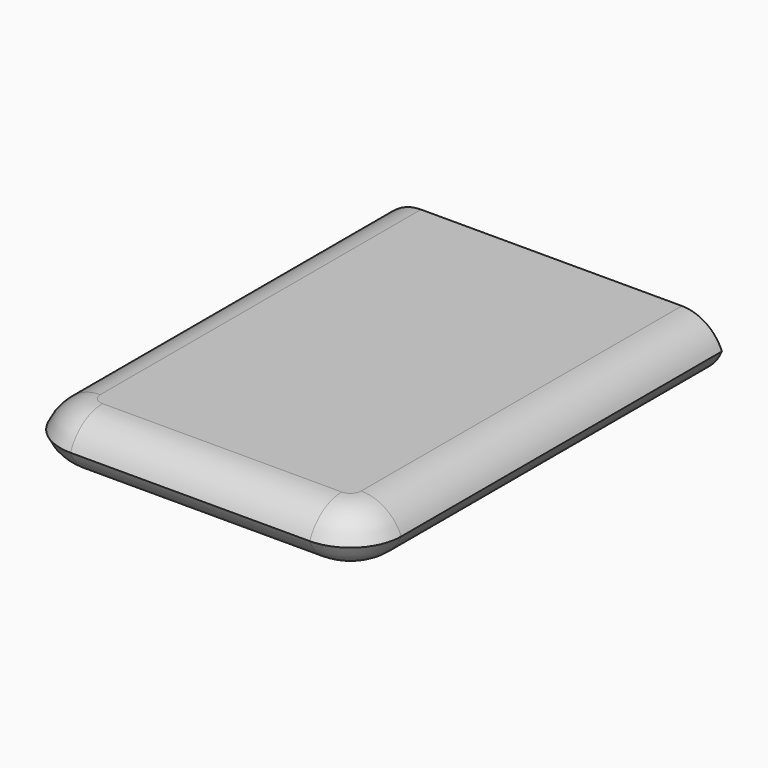
from build123d import *

# Parameters (mm, degrees)
F1_DEPTH     = 6.35
F2_T1_DEPTH  = 59.8574546933
F2_T3_DEPTH  = 28.1503971994
F2_T6_ANGLE  = 90
F2_T8_ANGLE  = 90
F2_T10_ANGLE = 90
F2_T12_ANGLE = 90


# Not quite as in the source:
# - a fillet or chamfer that OpenCascade refuses, or shapes differently, is made with other operations: its cross-section is extruded or revolved along the edge and cut away or added


with BuildPart() as f1:
    # F0 (on Top) → F1 (new body)
    with BuildSketch(Plane.XY):
        with BuildLine():
            Line((20.4174276441, 0), (-20.4329695553, 0))
            Line((-20.4329695553, 0), (-20.4329695553, -47.1574546933))
            ThreePointArc((-20.4329695553, -47.1574546933), (-18.5730976158, -51.6475827539), (-14.0829695553, -53.5074546933))
            Line((-14.0829695553, -53.5074546933), (14.0674276441, -53.5074546933))
            ThreePointArc((14.0674276441, -53.5074546933), (18.5575557047, -51.6475827539), (20.4174276441, -47.1574546933))
            Line((20.4174276441, -47.1574546933), (20.4174276441, 0))
        make_face()
    extrude(amount=F1_DEPTH)

    # F2: fillet of radius 5.08 on 10 edges, made by hand

    # F2_s2 → F2_t1 (cut)
    with BuildSketch(Plane.XZ.offset(-12.7)):
        with BuildLine():
            ThreePointArc((20.4174276441, 1.27), (18.9295300926, 4.8621024484), (15.3374276441, 6.35))
            Line((15.3374276441, 6.35), (20.4174276441, 6.35))
            Line((20.4174276441, 6.35), (20.4174276441, 1.27))
        make_face()
        with BuildLine():
            ThreePointArc((20.4174276441, 5.08), (18.9295300926, 1.4878975516), (15.3374276441, 0))
            Line((15.3374276441, 0), (20.4174276441, 0))
            Line((20.4174276441, 0), (20.4174276441, 5.08))
        make_face()
        with BuildLine():
            ThreePointArc((-20.4329695553, 1.27), (-18.9450720037, 4.8621024484), (-15.3529695553, 6.35))
            Line((-15.3529695553, 6.35), (-20.4329695553, 6.35))
            Line((-20.4329695553, 6.35), (-20.4329695553, 1.27))
        make_face()
        with BuildLine():
            ThreePointArc((-20.4329695553, 5.08), (-18.9450720037, 1.4878975516), (-15.3529695553, 0))
            Line((-15.3529695553, 0), (-20.4329695553, 0))
            Line((-20.4329695553, 0), (-20.4329695553, 5.08))
        make_face()
    extrude(amount=F2_T1_DEPTH, mode=Mode.SUBTRACT)

    # F2_s4 → F2_t3 (cut)
    with BuildSketch(Plane.YZ.offset(-14.0829695553)):
        with BuildLine():
            ThreePointArc((-53.5074546933, 5.08), (-52.0195571417, 1.4878975516), (-48.4274546933, 0))
            Line((-48.4274546933, 0), (-53.5074546933, 0))
            Line((-53.5074546933, 0), (-53.5074546933, 5.08))
        make_face()
        with BuildLine():
            ThreePointArc((-53.5074546933, 1.27), (-52.0195571417, 4.8621024484), (-48.4274546933, 6.35))
            Line((-48.4274546933, 6.35), (-53.5074546933, 6.35))
            Line((-53.5074546933, 6.35), (-53.5074546933, 1.27))
        make_face()
    extrude(amount=F2_T3_DEPTH, mode=Mode.SUBTRACT)

    # F2_s5 → F2_t6 (revolve, cut)
    with BuildSketch(Plane.YZ.offset(14.0674276441)):
        with BuildLine():
            ThreePointArc((-53.5074546933, 1.27), (-52.0195571417, 4.8621024484), (-48.4274546933, 6.35))
            Line((-48.4274546933, 6.35), (-53.5074546933, 6.35))
            Line((-53.5074546933, 6.35), (-53.5074546933, 1.27))
        make_face()
    revolve(axis=Axis((14.0674276441, -47.1574546933, 6.35), (0, 0, 1)), revolution_arc=F2_T6_ANGLE, mode=Mode.SUBTRACT)

    # F2_s7 → F2_t8 (revolve, cut)
    with BuildSketch(Plane.YZ.offset(14.0674276441)):
        with BuildLine():
            ThreePointArc((-53.5074546933, 5.08), (-52.0195571417, 1.4878975516), (-48.4274546933, 0))
            Line((-48.4274546933, 0), (-53.5074546933, 0))
            Line((-53.5074546933, 0), (-53.5074546933, 5.08))
        make_face()
    revolve(axis=Axis((14.0674276441, -47.1574546933, 0), (0, 0, 1)), revolution_arc=F2_T8_ANGLE, mode=Mode.SUBTRACT)

    # F2_s9 → F2_t10 (revolve, cut)
    with BuildSketch(Plane.XZ.offset(47.1574546933)):
        with BuildLine():
            ThreePointArc((-20.4329695553, 1.27), (-18.9450720037, 4.8621024484), (-15.3529695553, 6.35))
            Line((-15.3529695553, 6.35), (-20.4329695553, 6.35))
            Line((-20.4329695553, 6.35), (-20.4329695553, 1.27))
        make_face()
    revolve(axis=Axis((-14.0829695553, -47.1574546933, 6.35), (0, 0, 1)), revolution_arc=F2_T10_ANGLE, mode=Mode.SUBTRACT)

    # F2_s11 → F2_t12 (revolve, cut)
    with BuildSketch(Plane.XZ.offset(47.1574546933)):
        with BuildLine():
            ThreePointArc((-20.4329695553, 5.08), (-18.9450720037, 1.4878975516), (-15.3529695553, 0))
            Line((-15.3529695553, 0), (-20.4329695553, 0))
            Line((-20.4329695553, 0), (-20.4329695553, 5.08))
        make_face()
    revolve(axis=Axis((-14.0829695553, -47.1574546933, 0), (0, 0, 1)), revolution_arc=F2_T12_ANGLE, mode=Mode.SUBTRACT)


solid = f1.part
